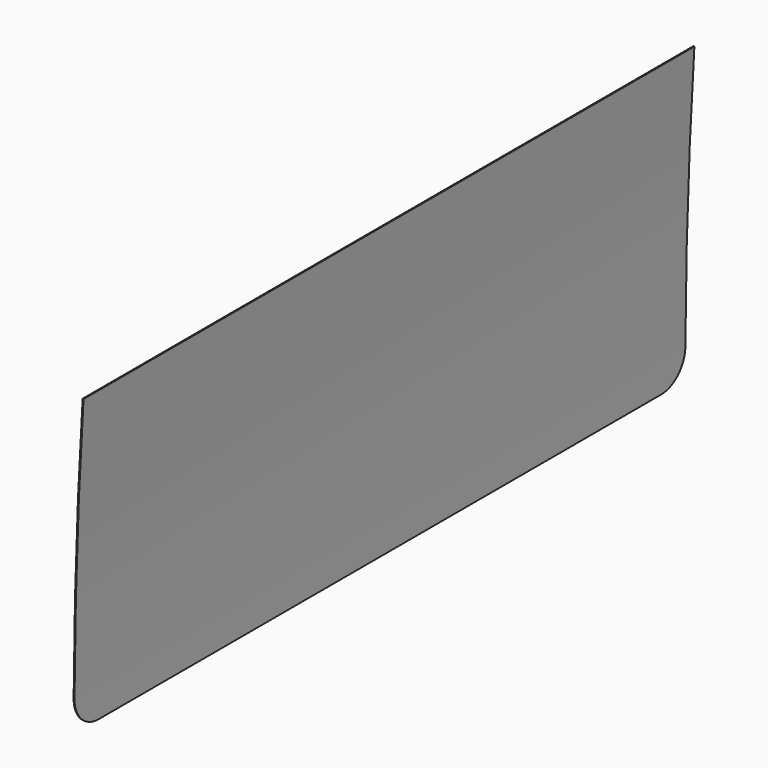
from build123d import *

# Parameters (mm, degrees)
F1_DEPTH = 2526
F2_R     = 100


with BuildPart() as f1:
    # F0 (on Front) → F1 (new body)
    with BuildSketch(Plane.XZ):
        with BuildLine():
            ThreePointArc((-685, 200), (-677.4536303253, 691.6975376497), (-654.8216297668, 1182.9319102019))
            Line((-654.8216297668, 1182.9319102019), (-657.8159792684, 1183.1159511275))
            ThreePointArc((-657.8159792684, 1183.1159511275), (-680.4522173679, 691.7896014733), (-688, 200))
            Line((-688, 200), (-685, 200))
        make_face()
    extrude(amount=F1_DEPTH)

    # F2
    f2_edges = [f1.edges().sort_by_distance(p)[0] for p in [
        (-686.5, -2526, 200),
        (-686.5, 0, 200),
    ]]
    fillet(f2_edges, radius=F2_R)


solid = f1.part
